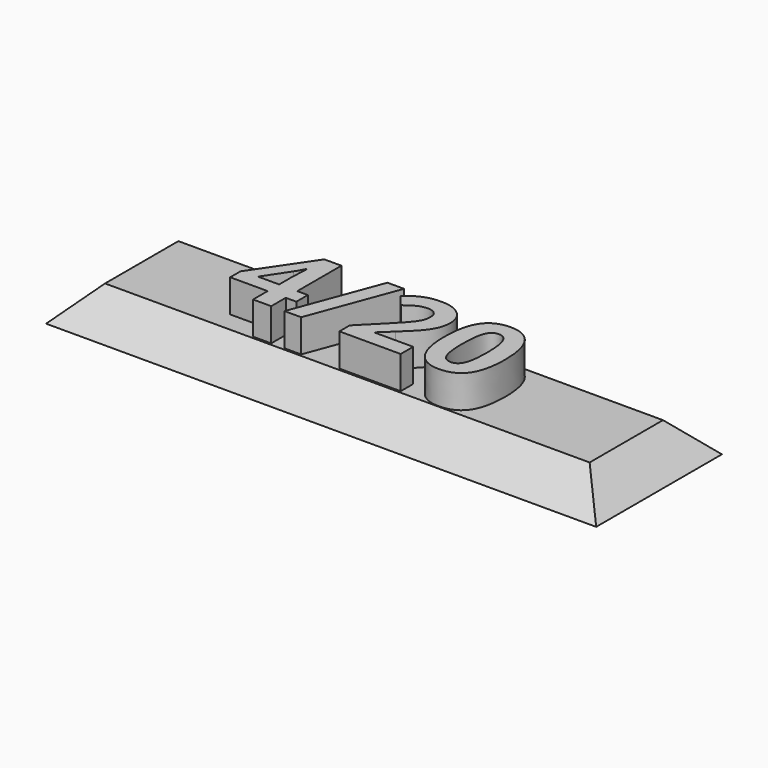
from build123d import *

# Parameters (mm, degrees)
F0_W         = 57.15
F0_H         = 19.05
F1_DEPTH     = 3.175
F2_T1_DEPTH  = 83.2782991577
F2_T3_DEPTH  = 45.1782991577
F3_TEXT_SIZE = 11.9156103918
F4_DEPTH     = 6.35


# Not quite as in the source:
# - a fillet or chamfer that OpenCascade refuses, or shapes differently, is made with other operations: its cross-section is extruded or revolved along the edge and cut away or added
# - Text() gives the source's letters only with a copy of the font that has no kerning and outlines rounded to 1/6400 em; it was checked with that copy


with BuildPart() as f1:
    # F0 (on Top) → F1 (new body)
    with BuildSketch(Plane.XY):
        with Locations((1.8937252462, -1.5693070905)):
            Rectangle(F0_W, F0_H)
    extrude(amount=F1_DEPTH)

    # F2: chamfer of 5.08 on 4 edges, made by hand

    # F2_s2 → F2_t1 (cut)
    with BuildSketch(Plane.YZ.offset(-39.7454243327)):
        Polygon((7.9556929095, -1.905), (2.8756929095, 3.175), (7.9556929095, 3.175), align=None)
        Polygon((-11.0943070905, -1.905), (-6.0143070905, 3.175), (-11.0943070905, 3.175), align=None)
    extrude(amount=F2_T1_DEPTH, mode=Mode.SUBTRACT)

    # F2_s4 → F2_t3 (cut)
    with BuildSketch(Plane.XZ.offset(-21.0198424884)):
        Polygon((-26.6812747538, -1.905), (-21.6012747538, 3.175), (-26.6812747538, 3.175), align=None)
        Polygon((30.4687252462, -1.905), (25.3887252462, 3.175), (30.4687252462, 3.175), align=None)
    extrude(amount=F2_T3_DEPTH, mode=Mode.SUBTRACT)

    # F3 (on Top) → F4 (join)
    with BuildSketch(Plane.XY):
        with Locations((-11.2290845718, -5.8255121112)):
            Text('4/20', F3_TEXT_SIZE, font='Open Sans', font_style=FontStyle.BOLD, text_align=(TextAlign.LEFT, TextAlign.BOTTOM))
    extrude(amount=F4_DEPTH)


solid = f1.part
